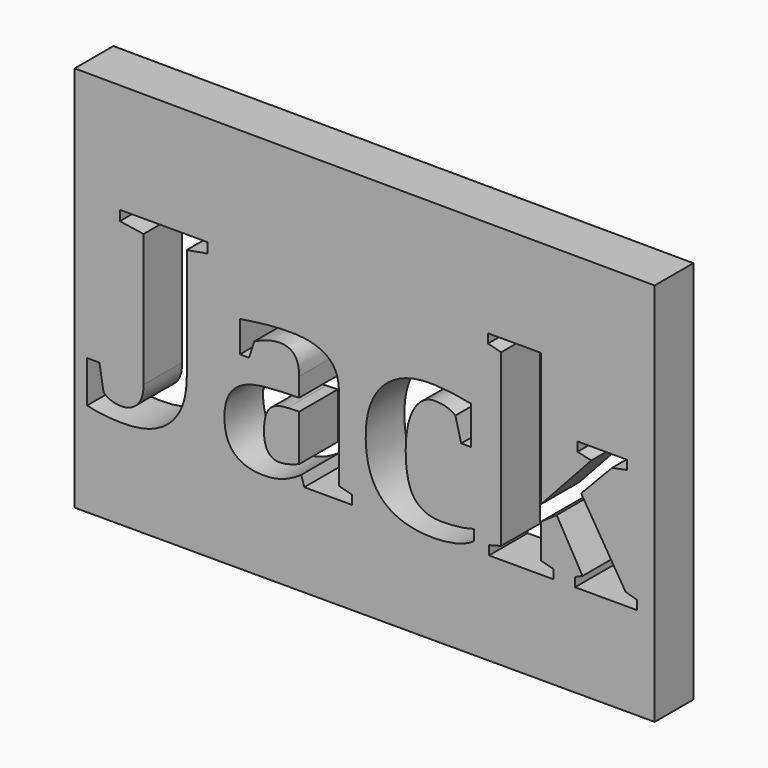
from build123d import *

# Parameters (mm, degrees)
F1_DEPTH     = 3.175
F2_TEXT_SIZE = 18.4853309074
F3_DEPTH     = 3.175


# Not quite as in the source:
# - Text() gives the source's letters only with a copy of the font that has no kerning and outlines rounded to 1/6400 em; it was checked with that copy


with BuildPart() as f1:
    # F0 (on Front) → F1 (new body)
    with BuildSketch(Plane.XZ):
        Polygon((0, 25.2371823891), (-38.0996521037, 25.4), (-38.0996521037, 0), (0, 0), align=None)
    extrude(amount=F1_DEPTH)

    # F2 (on face) → F3 (cut)
    with BuildSketch(Plane.XZ.offset(3.175)):
        with Locations((-38.0996521037, 6.0857441357)):
            Text('Jack', F2_TEXT_SIZE, font='Tinos', font_style=FontStyle.BOLD, text_align=(TextAlign.LEFT, TextAlign.BOTTOM))
    extrude(amount=-F3_DEPTH, mode=Mode.SUBTRACT)


solid = f1.part
